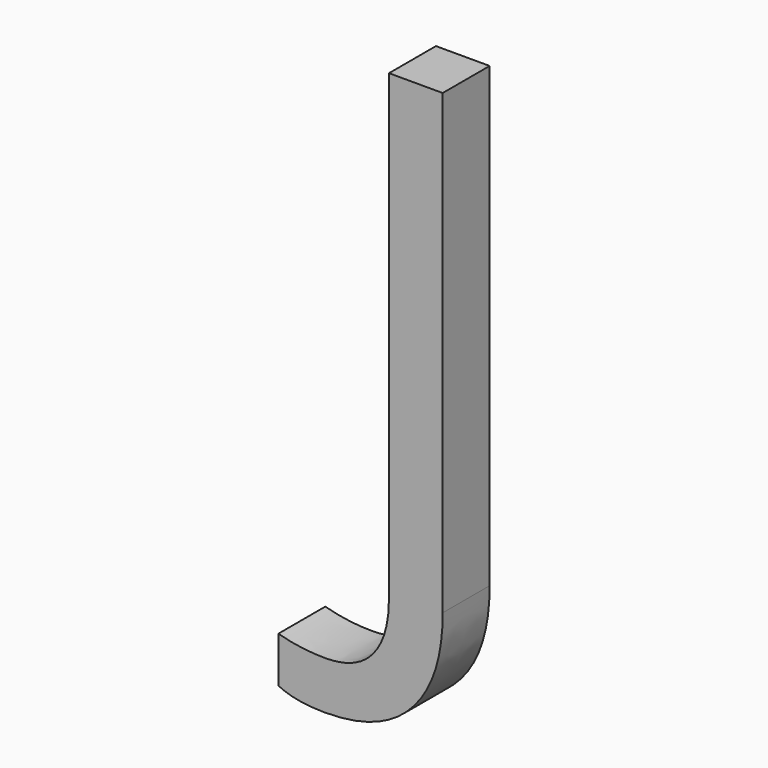
from build123d import *

# Parameters (mm, degrees)
F0_TEXT_SIZE = 140.0711066607
F1_DEPTH     = 12.7


# Not quite as in the source:
# - Text() gives the source's letters only with a copy of the font that has no kerning and outlines rounded to 1/6400 em; it was checked with that copy


with BuildPart() as f1:
    # F0 (on Front) → F1 (new body)
    with BuildSketch(Plane.XZ):
        with Locations((-18.3227881789, -42.9302155972)):
            Text('J', F0_TEXT_SIZE, font='Open Sans', text_align=(TextAlign.LEFT, TextAlign.BOTTOM))
    extrude(amount=F1_DEPTH)


solid = f1.part
